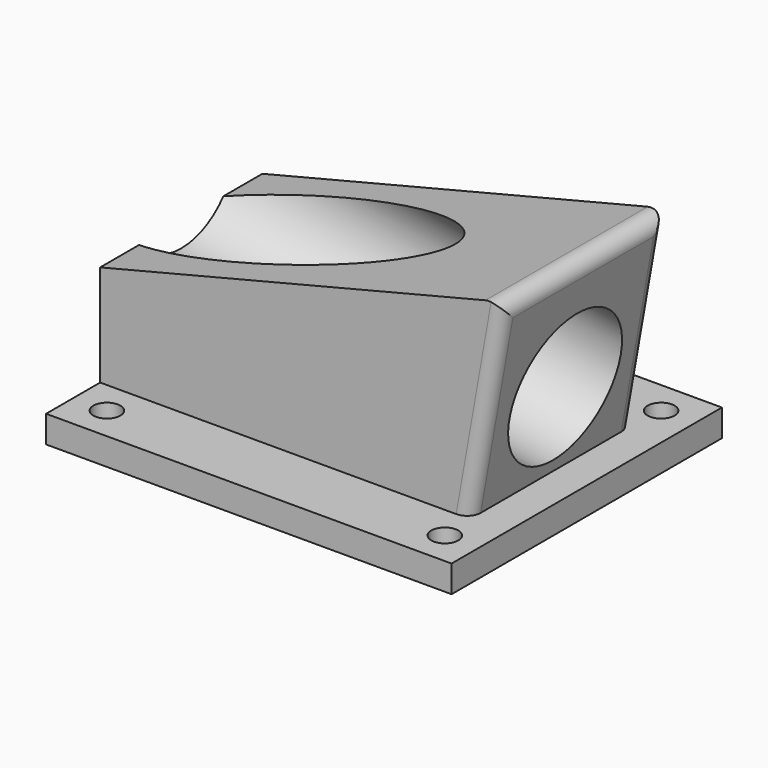
from build123d import *

# Parameters (mm, degrees)
F0_W      = 30
F0_H      = 25
F1_DEPTH  = 2
F2_R      = 1
F3_DEPTH  = 2
F4_W      = 30
F4_H      = 15
F5_DEPTH  = 15
F7_DEPTH  = 15
F9_DEPTH  = 15
F10_R     = 5.15
F11_DEPTH = 28.2428712579
F12_R     = 1


with BuildPart() as f1:
    # F0 (on Top) → F1 (new body)
    with BuildSketch(Plane.XY):
        Rectangle(F0_W, F0_H)
    extrude(amount=F1_DEPTH)

    # F2 (on face) → F3 (cut)
    with BuildSketch(Plane.XY.offset(2)):
        with Locations((12.5, 10)):
            Circle(F2_R)
        with Locations((-12.5, 10)):
            Circle(F2_R)
        with Locations((-12.5, -10)):
            Circle(F2_R)
        with Locations((12.5, -10)):
            Circle(F2_R)
    extrude(amount=-F3_DEPTH, mode=Mode.SUBTRACT)

    # F4 (on face) → F5 (join)
    with BuildSketch(Plane.XY.offset(2)):
        Rectangle(F4_W, F4_H)
    extrude(amount=F5_DEPTH)

    # F6 (on face) → F7 (cut, through all)
    with BuildSketch(Plane.XZ.offset(7.5)):
        Polygon((-15, 9.5), (15, 17), (-15, 17), align=None)
    extrude(amount=-F7_DEPTH, mode=Mode.SUBTRACT)

    # F8 (on face) → F9 (cut, through all)
    with BuildSketch(Plane.XZ.offset(7.5)):
        Polygon((15, 2), (15, 17), (12.3550952894, 2), align=None)
    extrude(amount=-F9_DEPTH, mode=Mode.SUBTRACT)

    # F10 (on face) → F11 (cut, through all)
    with BuildSketch(Plane(origin=(11.6405234376, 0, -2.0525383516), x_dir=(0, 1, 0), z_dir=(0.984807753, 0, -0.1736481777))):
        with Locations((0, 10.1150552879)):
            Circle(F10_R)
    extrude(amount=-F11_DEPTH, mode=Mode.SUBTRACT)

    # F12
    f12_edges = [f1.edges().sort_by_distance(p)[0] for p in [
        (13.677548, -7.5, 9.5),
        (13.677548, 7.5, 9.5),
        (15, 0, 17),
    ]]
    fillet(f12_edges, radius=F12_R)


solid = f1.part
